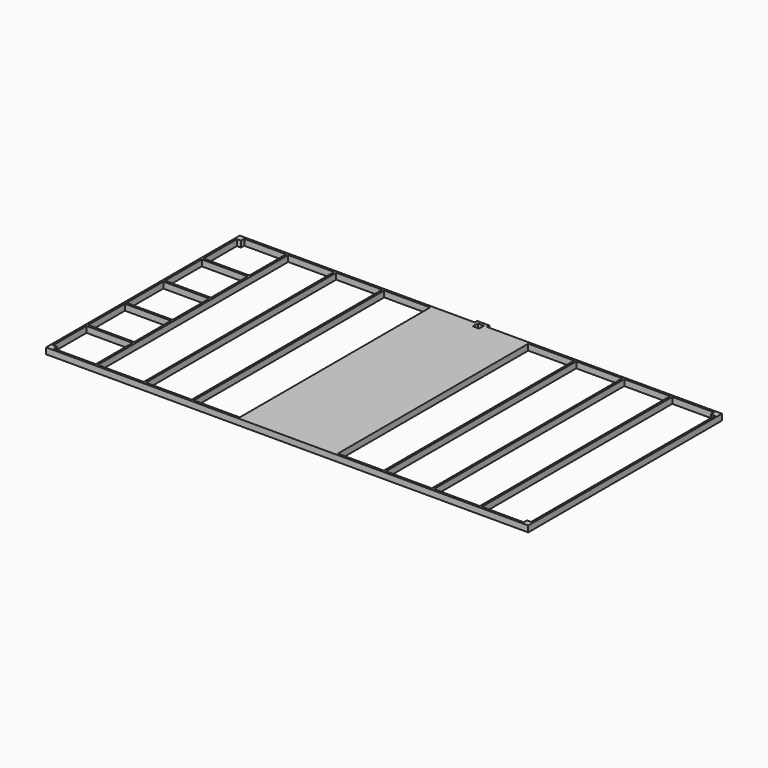
from build123d import *

# Parameters (mm, degrees)
F0_W     = 50.8
F0_H     = 5918.2
F0_W_2   = 1143
F0_H_2   = 50.8
F0_W_3   = 76.2
F0_H_3   = 5740.4
F0_H_4   = 76.2
F0_H_5   = 5715
F1_DEPTH = 152.4


# Not quite as in the source:
# - a feature names something its author has since deleted; it is built from what else it names


with BuildPart() as f1:
    # F0 (on Top) → F1 (new body)
    with BuildSketch(Plane.XY):
        Polygon((-1.9920532227, 5379.496395874), (1141.0079467773, 5379.496395874), (1191.8079467773, 5379.496395874), (2334.8079467773, 5379.496395874), (2385.6079467774, 5379.496395874), (3528.6079467773, 5379.496395874), (3579.4079467774, 5379.496395874), (4595.4079467774, 5379.496395874), (4595.4079467774, 5430.296395874), (-1094.1920532227, 5430.296395874), (-1094.1920532227, 5379.496395874), (-52.7920532227, 5379.496395874), align=None)
        with Locations((1166.4079467773, 2420.396395874)):
            Rectangle(F0_W, F0_H)
        Polygon((1191.8079467773, -538.703604126), (1141.0079467773, -538.703604126), (-1.9920532227, -538.703604126), (-52.7920532227, -538.703604126), (-1094.1920532227, -538.703604126), (-1094.1920532227, -589.503604126), (10589.8079467774, -589.503604126), (10589.8079467774, -538.703604126), (9548.4079467774, -538.703604126), (9497.6079467774, -538.703604126), (8354.6079467774, -538.703604126), (8303.8079467774, -538.703604126), (7160.8079467774, -538.703604126), (7110.0079467774, -538.703604126), (5967.0079467774, -538.703604126), (5916.2079467774, -538.703604126), (4773.2079467774, -538.703604126), (4722.4079467774, -538.703604126), (3579.4079467774, -538.703604126), (3528.6079467774, -538.703604126), (2385.6079467774, -538.703604126), (2334.8079467773, -538.703604126), align=None)
        Polygon((-1.9920532227, -538.703604126), (-1.9920532227, 5379.496395874), (-52.7920532227, 5379.496395874), (-52.7920532227, 4236.496395874), (-52.7920532227, 4185.696395874), (-52.7920532227, 3042.696395874), (-52.7920532227, 2991.896395874), (-52.7920532227, 1848.896395874), (-52.7920532227, 1798.096395874), (-52.7920532227, 655.096395874), (-52.7920532227, 604.296395874), (-52.7920532227, -538.703604126), align=None)
        with Locations((2360.2079467773, 2420.396395874)):
            Rectangle(F0_W, F0_H)
        with Locations((-624.2920532227, 4211.096395874)):
            Rectangle(F0_W_2, F0_H_2)
        Polygon((-1094.1920532227, 5277.896395874), (-1094.1920532227, 5379.496395874), (-1094.1920532227, 5430.296395874), (-1246.5920532227, 5430.296395874), (-1246.5920532227, 5277.896395874), (-1195.7920532227, 5277.896395874), align=None)
        with Locations((3554.0079467774, 2420.396395874)):
            Rectangle(F0_W, F0_H)
        with Locations((-624.2920532227, 629.696395874)):
            Rectangle(F0_W_2, F0_H_2)
        Polygon((-1094.1920532227, -589.503604126), (-1094.1920532227, -538.703604126), (-1094.1920532227, -437.103604126), (-1195.7920532227, -437.103604126), (-1246.5920532227, -437.103604126), (-1246.5920532227, -589.503604126), align=None)
        Polygon((-1195.7920532227, 4185.696395874), (-1195.7920532227, 4236.496395874), (-1195.7920532227, 5277.896395874), (-1246.5920532227, 5277.896395874), (-1246.5920532227, -437.103604126), (-1195.7920532227, -437.103604126), (-1195.7920532227, 604.296395874), (-1195.7920532227, 655.096395874), (-1195.7920532227, 1798.096395874), (-1195.7920532227, 1848.896395874), (-1195.7920532227, 2991.896395874), (-1195.7920532227, 3042.696395874), align=None)
        Polygon((4595.4079467774, 5379.496395874), (3579.4079467774, 5379.496395874), (3579.4079467774, -538.703604126), (4722.4079467774, -538.703604126), (4722.4079467774, 5201.696395874), (4595.4079467774, 5201.696395874), align=None)
        with Locations((-624.2920532227, 3017.296395874)):
            Rectangle(F0_W_2, F0_H_2)
        Polygon((4595.4079467774, 5506.496395874), (4595.4079467774, 5430.296395874), (4671.6079467774, 5430.296395874), (4824.0079467774, 5430.296395874), (4900.2079467774, 5430.296395874), (4900.2079467774, 5506.496395874), align=None)
        with Locations((4633.5079467774, 5404.896395874)):
            Rectangle(F0_W_3, F0_H_2)
        Polygon((4671.6079467774, 5379.496395874), (4595.4079467774, 5379.496395874), (4595.4079467774, 5201.696395874), (4722.4079467774, 5201.696395874), (4722.4079467774, 5277.896395874), (4671.6079467774, 5277.896395874), align=None)
        with Locations((-624.2920532227, 1823.496395874)):
            Rectangle(F0_W_2, F0_H_2)
        Polygon((10589.8079467774, -538.703604126), (10589.8079467774, -589.503604126), (10742.2079467774, -589.503604126), (10742.2079467774, -437.103604126), (10691.4079467774, -437.103604126), (10589.8079467774, -437.103604126), align=None)
        with Locations((4747.8079467774, 2331.496395874)):
            Rectangle(F0_W, F0_H_3)
        with Locations((4862.1079467774, 5404.896395874)):
            Rectangle(F0_W_3, F0_H_2)
        Polygon((4773.2079467774, 5201.696395874), (4773.2079467774, -538.703604126), (5916.2079467774, -538.703604126), (5916.2079467774, 5379.496395874), (4900.2079467774, 5379.496395874), (4900.2079467774, 5201.696395874), align=None)
        with Locations((4747.8079467774, 5239.796395874)):
            Rectangle(F0_W, F0_H_4)
        with Locations((9523.0079467774, 2420.396395874)):
            Rectangle(F0_W, F0_H)
        with Locations((10716.8079467774, 2420.396395874)):
            Rectangle(F0_W, F0_H_5)
        Polygon((10589.8079467774, 5430.296395874), (4900.2079467774, 5430.296395874), (4900.2079467774, 5379.496395874), (5916.2079467774, 5379.496395874), (5967.0079467774, 5379.496395874), (7110.0079467774, 5379.496395874), (7160.8079467774, 5379.496395874), (8303.8079467774, 5379.496395874), (8354.6079467774, 5379.496395874), (9497.6079467774, 5379.496395874), (9548.4079467774, 5379.496395874), (10589.8079467774, 5379.496395874), align=None)
        Polygon((4900.2079467774, 5379.496395874), (4824.0079467774, 5379.496395874), (4824.0079467774, 5277.896395874), (4773.2079467774, 5277.896395874), (4773.2079467774, 5201.696395874), (4900.2079467774, 5201.696395874), align=None)
        with Locations((5941.6079467774, 2420.396395874)):
            Rectangle(F0_W, F0_H)
        Polygon((10691.4079467774, 5277.896395874), (10742.2079467774, 5277.896395874), (10742.2079467774, 5430.296395874), (10589.8079467774, 5430.296395874), (10589.8079467774, 5379.496395874), (10589.8079467774, 5277.896395874), align=None)
        with Locations((8329.2079467774, 2420.396395874)):
            Rectangle(F0_W, F0_H)
        with Locations((7135.4079467774, 2420.396395874)):
            Rectangle(F0_W, F0_H)
    extrude(amount=F1_DEPTH)


solid = f1.part
